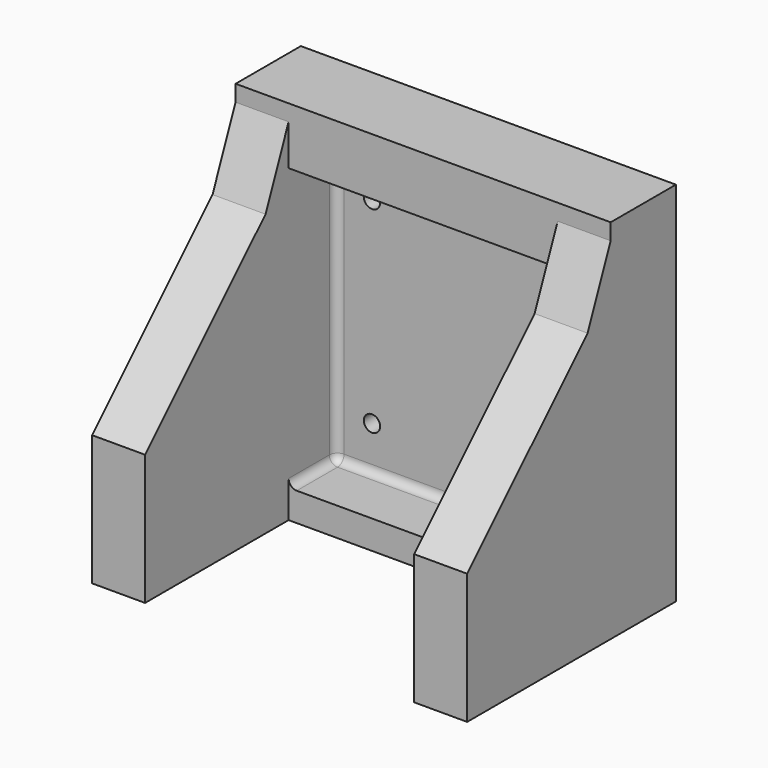
from build123d import *

# Parameters (mm, degrees)
F0_W      = 32
F0_H      = 42
F1_DEPTH  = 46
F2_W      = 33
F2_H      = 29.25
F3_DEPTH  = 42.001
F4_SIZE   = 26
F5_R      = 1
F6_DEPTH  = 25
F7_W      = 46
F7_H      = 7
F7_H_2    = 3.5
F8_DEPTH  = 10
F9_SIZE   = 5
F10_R     = 1
F11_R     = 0.75
F12_DEPTH = 5


with BuildPart() as f1:
    # F0 (on Right) → F1 (new body)
    with BuildSketch(Plane.YZ):
        with Locations((16, 21)):
            Rectangle(F0_W, F0_H)
    extrude(amount=-F1_DEPTH)

    # F2 (on Top) → F3 (cut, through all)
    with BuildSketch(Plane.XY):
        with Locations((-23, 14.625)):
            Rectangle(F2_W, F2_H)
    extrude(amount=F3_DEPTH, mode=Mode.SUBTRACT)

    # F4
    f4_edges = [f1.edges().sort_by_distance(p)[0] for p in [
        (-42.75, 0, 42),
        (-3.25, 0, 42),
    ]]
    chamfer(f4_edges, length=F4_SIZE)

    # F5 (on face) → F6 (cut)
    with BuildSketch(Plane.XZ.offset(-29.25)):
        with Locations((-35.0738482888, 33.0738482888)):
            Circle(F5_R)
        with Locations((-10.9261517112, 33.0738482888)):
            Circle(F5_R)
        with Locations((-35.0738482888, 8.9261517112)):
            Circle(F5_R)
        with Locations((-10.9261517112, 8.9261517112)):
            Circle(F5_R)
    extrude(amount=-F6_DEPTH, mode=Mode.SUBTRACT)

    # F7 (on face) → F8 (join)
    with BuildSketch(Plane(origin=(0, 32, 0), x_dir=(-1, 0, 0), z_dir=(0, 1, 0))):
        with Locations((23, 41.5)):
            Rectangle(F7_W, F7_H)
        with Locations((23, 1.75)):
            Rectangle(F7_W, F7_H_2)
    extrude(amount=-F8_DEPTH)

    # F9
    f9_edges = [f1.edges().sort_by_distance(p)[0] for p in [
        (-42.75, 22, 38),
        (-3.25, 22, 38),
    ]]
    chamfer(f9_edges, length=F9_SIZE)

    # F10
    f10_edges = [f1.edges().sort_by_distance(p)[0] for p in [
        (-39.5, 29.25, 20.75),
        (-6.5, 29.25, 20.75),
        (-23, 29.25, 38),
        (-23, 29.25, 3.5),
        (-39.5, 25.625, 3.5),
        (-6.5, 25.625, 3.5),
    ]]
    fillet(f10_edges, radius=F10_R)

    # F11 (on face) → F12 (cut)
    with BuildSketch(Plane(origin=(0, 0, 0), x_dir=(1, 0, 0), z_dir=(0, 0, -1))):
        with Locations((-42.75, -4)):
            Circle(F11_R)
        with Locations((-42.75, -28.5)):
            Circle(F11_R)
        with Locations((-3.25, -28.5)):
            Circle(F11_R)
        with Locations((-3.25, -4)):
            Circle(F11_R)
    extrude(amount=-F12_DEPTH, mode=Mode.SUBTRACT)


solid = f1.part
